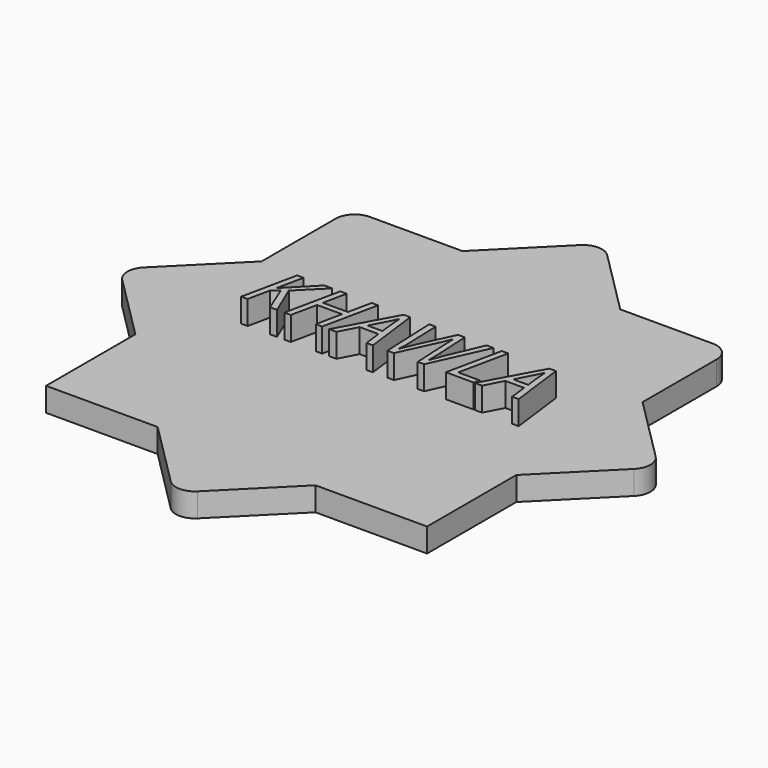
from build123d import *

# Parameters (mm, degrees)
F1_DEPTH     = 2.5
F3_TEXT_SIZE = 8.1314585804
F4_DEPTH     = 2.5


# Not quite as in the source:
# - Text() gives the source's letters only with a copy of the font that has no kerning and outlines rounded to 1/6400 em; it was checked with that copy


with BuildPart() as f1:
    # F0 (on Top) → F1 (new body)
    with BuildSketch(Plane.XY):
        Polygon((8.2842712475, -20), (20, -20), (20, -8.2842712475), align=None)
        with BuildLine():
            Line((1.4142135624, -26.8700576851), (8.2842712475, -20))
            Line((8.2842712475, -20), (-8.2842712475, -20))
            Line((-8.2842712475, -20), (-1.4142135624, -26.8700576851))
            ThreePointArc((-1.4142135624, -26.8700576851), (0, -27.4558441227), (1.4142135624, -26.8700576851))
        make_face()
        Polygon((-8.2842712475, -20), (8.2842712475, -20), (20, -8.2842712475), (20, 8.2842712475), (8.2842712475, 20), (-8.2842712475, 20), (-20, 8.2842712475), (-20, -8.2842712475), align=None)
        with BuildLine():
            Line((20, 8.2842712475), (20, -8.2842712475))
            Line((20, -8.2842712475), (26.8700576851, -1.4142135624))
            ThreePointArc((26.8700576851, -1.4142135624), (27.4558441227, 0), (26.8700576851, 1.4142135624))
            Line((26.8700576851, 1.4142135624), (20, 8.2842712475))
        make_face()
        Polygon((-20, -20), (-8.2842712475, -20), (-20, -8.2842712475), align=None)
        with BuildLine():
            Line((8.2842712475, 20), (20, 8.2842712475))
            Line((20, 8.2842712475), (20, 18))
            ThreePointArc((20, 18), (19.4142135624, 19.4142135624), (18, 20))
            Line((18, 20), (8.2842712475, 20))
        make_face()
        with BuildLine():
            Line((-26.8700576851, -1.4142135624), (-20, -8.2842712475))
            Line((-20, -8.2842712475), (-20, 8.2842712475))
            Line((-20, 8.2842712475), (-26.8700576851, 1.4142135624))
            ThreePointArc((-26.8700576851, 1.4142135624), (-27.4558441227, 0), (-26.8700576851, -1.4142135624))
        make_face()
        with BuildLine():
            Line((-8.2842712475, 20), (8.2842712475, 20))
            Line((8.2842712475, 20), (1.4142135624, 26.8700576851))
            ThreePointArc((1.4142135624, 26.8700576851), (0, 27.4558441227), (-1.4142135624, 26.8700576851))
            Line((-1.4142135624, 26.8700576851), (-8.2842712475, 20))
        make_face()
        with BuildLine():
            Line((-20, 18), (-20, 8.2842712475))
            Line((-20, 8.2842712475), (-8.2842712475, 20))
            Line((-8.2842712475, 20), (-18, 20))
            ThreePointArc((-18, 20), (-19.4142135624, 19.4142135624), (-20, 18))
        make_face()
    extrude(amount=F1_DEPTH)

    # F3 (on face) → F4 (join)
    with BuildSketch(Plane.XY.offset(2.5)):
        with Locations((-14.7389497608, -1.3987644403)):
            Text('KHAWLA', F3_TEXT_SIZE, font='Open Sans', font_style=FontStyle.ITALIC, text_align=(TextAlign.LEFT, TextAlign.BOTTOM))
    extrude(amount=F4_DEPTH)


solid = f1.part
